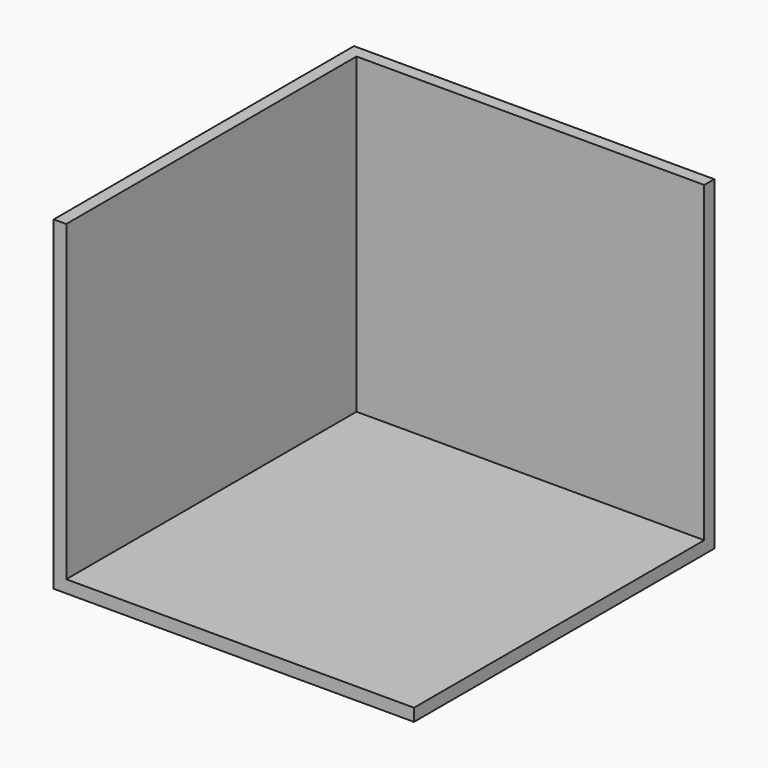
from build123d import *

# Parameters (mm, degrees)
F0_W     = 100
F0_H     = 2600
F1_DEPTH = 3000
F2_W     = 100
F2_H     = 2600
F3_DEPTH = 2780
F4_W     = 2780
F4_H     = 2900
F5_DEPTH = 100


with BuildPart() as f1:
    # F0 (on Front) → F1 (new body)
    with BuildSketch(Plane.XZ):
        with Locations((50, 1300)):
            Rectangle(F0_W, F0_H)
    extrude(amount=F1_DEPTH)

    # F2 (on face) → F3 (join)
    with BuildSketch(Plane.YZ.offset(100)):
        with Locations((-50, 1300)):
            Rectangle(F2_W, F2_H)
    extrude(amount=F3_DEPTH)

    # F4 (on face) → F5 (join)
    with BuildSketch(Plane(origin=(0, 0, 0), x_dir=(1, 0, 0), z_dir=(0, 0, -1))):
        Polygon((100, 3000), (0, 3000), (0, 0), (2880, 0), (2880, 100), (100, 100), align=None)
        with Locations((1490, 1550)):
            Rectangle(F4_W, F4_H)
    extrude(amount=-F5_DEPTH)


solid = f1.part
